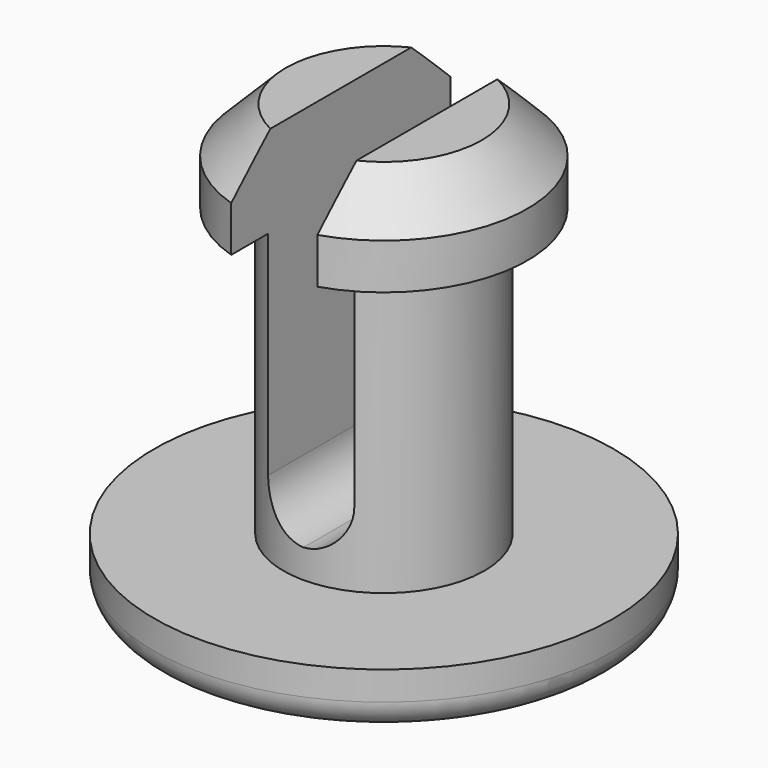
from build123d import *

# Parameters (mm, degrees)
F2_SIZE       = 0.79375
F3_W          = 1.5
F3_H          = 6.0875
F4_DEPTH      = 4.001
F4_DEPTH_BACK = 4.001
F5_T4_DEPTH   = 7.1310276602
F5_S5_R       = 1.75
F5_T6_DEPTH   = 5
F5_T10_DEPTH  = 7.1310276602
F5_S11_R      = 1.75
F5_T12_DEPTH  = 5
F6_R          = 0.5


# Not quite as in the source:
# - a fillet or chamfer that OpenCascade refuses, or shapes differently, is made with other operations: its cross-section is extruded or revolved along the edge and cut away or added


with BuildPart() as f1:
    # F0 (on Front) → F1 (revolve)
    with BuildSketch(Plane.XZ):
        Polygon((4, 0), (1.75, 0), (1.75, 5), (2.5, 5), (2.5, 6.5875), (0, 6.5875), (0, 5), (0, 0), (0, -1), (4, -1), align=None)
    revolve(axis=Axis((0, 0, 2.5), (0, 0, 1)))

    # F2
    f2_edges = [f1.edges().sort_by_distance(p)[0] for p in [
        (-2.5, 0, 6.5875),
    ]]
    chamfer(f2_edges, length=F2_SIZE)

    # F3 (on Front) → F4 (cut, two sides)
    with BuildSketch(Plane.XZ) as f4_sk:
        with Locations((0, 3.54375)):
            Rectangle(F3_W, F3_H)
    extrude(amount=F4_DEPTH, mode=Mode.SUBTRACT)
    extrude(f4_sk.sketch, amount=-F4_DEPTH_BACK, mode=Mode.SUBTRACT)

    # F5: fillet of radius 0.79375 on 2 edges, made by hand


with BuildPart() as f5_tool2:
    # F5_s3 → F5_t4 (new body)
    with BuildSketch(Plane.XZ.offset(-3.5655138301)):
        with BuildLine():
            ThreePointArc((-0.04375, 0.5), (0.5175160076, 0.7324839924), (0.75, 1.29375))
            Line((0.75, 1.29375), (0.75, 0.5))
            Line((0.75, 0.5), (-0.04375, 0.5))
        make_face()
    extrude(amount=F5_T4_DEPTH)

    # F5_s5 → F5_t6 (intersect, symmetric)
    with BuildSketch(Plane.XY.offset(0.9)):
        Circle(F5_S5_R)
    extrude(amount=F5_T6_DEPTH, both=True, mode=Mode.INTERSECT)


with BuildPart() as f1_1:
    add(f1.part)

    # F5_t1: union F5_tool2
    add(f5_tool2.part)


with BuildPart() as f5_tool8:
    # F5_s9 → F5_t10 (new body)
    with BuildSketch(Plane.XZ.offset(-3.5655138301)):
        with BuildLine():
            ThreePointArc((-0.75, 1.29375), (-0.5175160076, 0.7324839924), (0.04375, 0.5))
            Line((0.04375, 0.5), (-0.75, 0.5))
            Line((-0.75, 0.5), (-0.75, 1.29375))
        make_face()
    extrude(amount=F5_T10_DEPTH)

    # F5_s11 → F5_t12 (intersect, symmetric)
    with BuildSketch(Plane.XY.offset(0.9)):
        Circle(F5_S11_R)
    extrude(amount=F5_T12_DEPTH, both=True, mode=Mode.INTERSECT)


with BuildPart() as f1_2:
    add(f1_1.part)

    # F5_t7: union F5_tool8
    add(f5_tool8.part)

    # F6
    f6_edges = [f1_2.edges().sort_by_distance(p)[0] for p in [
        (-4, 0, -1),
    ]]
    fillet(f6_edges, radius=F6_R)


solid = f1_2.part
